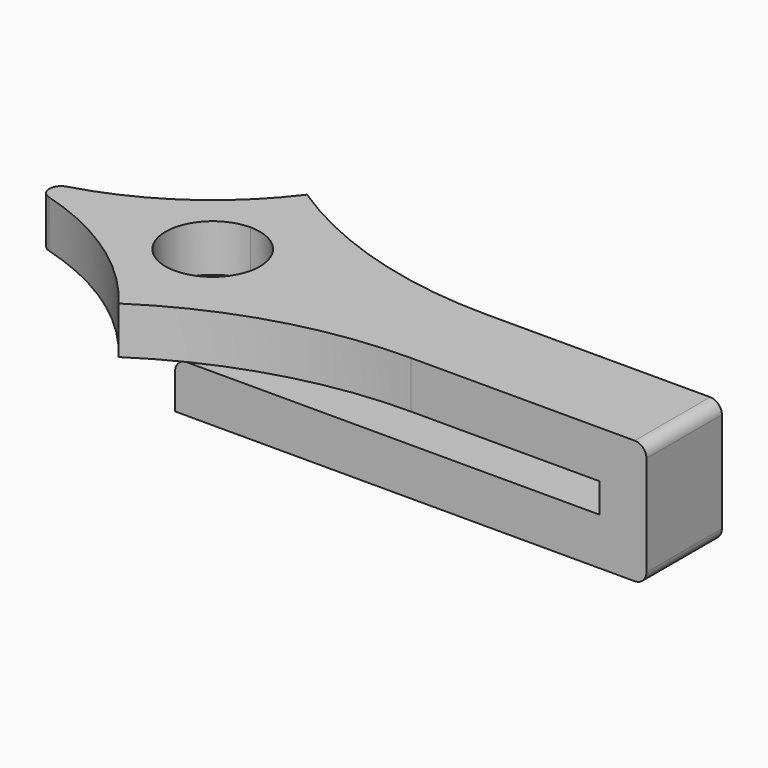
from build123d import *

# Parameters (mm, degrees)
F4_DEPTH = 2
F5_DEPTH = 1.25
F6_START = -1.25
F6_DEPTH = 2
F8_DEPTH = 4


# Not quite as in the source:
# - a feature names something its author has since deleted; it is built from what else it names


with BuildPart() as f4:
    # F3 (on Top) → F4 (new body)
    with BuildSketch(Plane.XY):
        with BuildLine():
            Line((0, -2), (0, 0))
            Line((0, 0), (0, 2))
            Line((0, 2), (-8, 2))
            Line((-8, 2), (-18, 2))
            ThreePointArc((-18, 2), (-16.5857864376, 1.4142135624), (-16, 0))
            ThreePointArc((-16, 0), (-16.5857864376, -1.4142135624), (-18, -2))
            Line((-18, -2), (-8, -2))
            Line((-8, -2), (0, -2))
        make_face()
        Polygon((0, 2), (0, 0), (0, -2), (2, -2), (2, 2), align=None)
        with BuildLine():
            Line((-18, 2), (-8, 2))
            ThreePointArc((-8, 2), (-13.2201532545, 2.7661558185), (-18, 5))
            ThreePointArc((-18, 5), (-20.9134084444, 2.2029023447), (-24.5666209478, 0.4807692308))
            ThreePointArc((-24.5666209478, 0.4807692308), (-24.9292857857, 0), (-24.5666209478, -0.4807692308))
            ThreePointArc((-24.5666209478, -0.4807692308), (-20.9134084444, -2.2029023447), (-18, -5))
            ThreePointArc((-18, -5), (-13.2201532545, -2.7661558185), (-8, -2))
            Line((-8, -2), (-18, -2))
            ThreePointArc((-18, -2), (-20, 0), (-18, 2))
        make_face()
    extrude(amount=F4_DEPTH)

    # F3 (on Top) → F5 (join)
    with BuildSketch(Plane.XY):
        Polygon((0, 2), (0, 0), (0, -2), (2, -2), (2, 2), align=None)
    extrude(amount=-F5_DEPTH)

    # F3 (on Top) → F6 (join)
    with BuildSketch(Plane.XY.offset(F6_START)):
        with BuildLine():
            Line((0, -2), (0, 0))
            Line((0, 0), (0, 2))
            Line((0, 2), (-8, 2))
            Line((-8, 2), (-18, 2))
            ThreePointArc((-18, 2), (-16.5857864376, 1.4142135624), (-16, 0))
            ThreePointArc((-16, 0), (-16.5857864376, -1.4142135624), (-18, -2))
            Line((-18, -2), (-8, -2))
            Line((-8, -2), (0, -2))
        make_face()
        Polygon((0, 2), (0, 0), (0, -2), (2, -2), (2, 2), align=None)
        with BuildLine():
            ThreePointArc((-16, 0), (-16.5857864376, 1.4142135624), (-18, 2))
            Line((-18, 2), (-18, -2))
            ThreePointArc((-18, -2), (-16.5857864376, -1.4142135624), (-16, 0))
        make_face()
    extrude(amount=-F6_DEPTH)

    # F7 (on face) → F8 (cut)
    with BuildSketch(Plane.XZ.offset(2)):
        with BuildLine():
            Line((-18, -1.25), (-18, -1.75))
            ThreePointArc((-18, -1.75), (-17.8535533906, -1.3964466094), (-17.5, -1.25))
            Line((-17.5, -1.25), (-18, -1.25))
        make_face()
        with BuildLine():
            ThreePointArc((1.5, 2), (1.8535533906, 1.8535533906), (2, 1.5))
            Line((2, 1.5), (2, 2))
            Line((2, 2), (1.5, 2))
        make_face()
        with BuildLine():
            ThreePointArc((2, -2.75), (1.8535533906, -3.1035533906), (1.5, -3.25))
            Line((1.5, -3.25), (2, -3.25))
            Line((2, -3.25), (2, -2.75))
        make_face()
    extrude(amount=-F8_DEPTH, mode=Mode.SUBTRACT)


solid = f4.part
